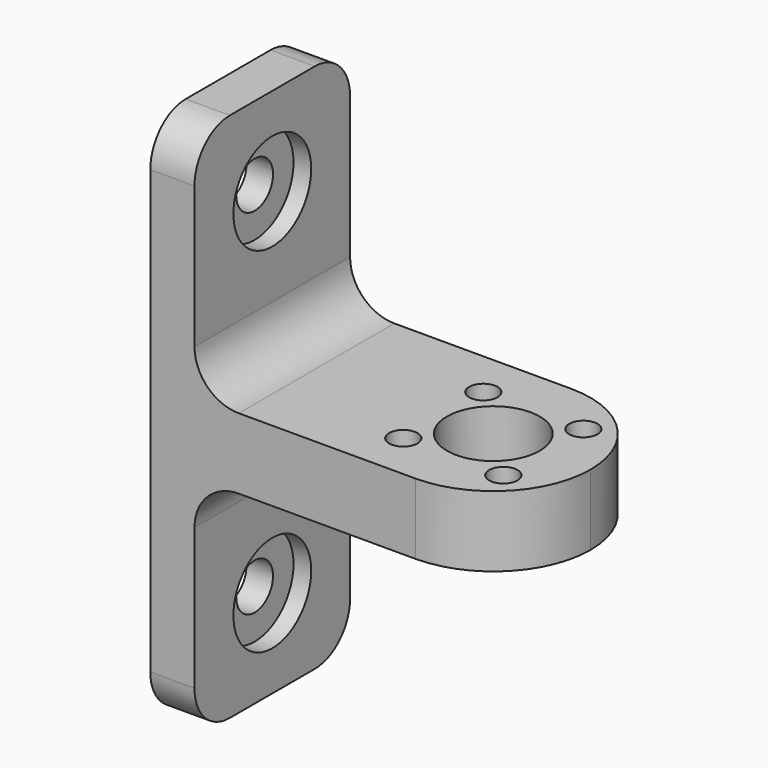
from build123d import *

# Parameters (mm, degrees)
F1_W            = 22
F1_H            = 26
F1_H_2          = 8
F2_DEPTH        = 5
F3_DEPTH        = 41
F5_D            = 10.5
F6_D            = 3.2
F7_R            = 10.99999
F8_R            = 5
F10_D           = 5.2
F10_CBORE_D     = 11
F10_CBORE_DEPTH = 2
F11_R           = 5


# Not quite as in the source:
# - a fillet or chamfer is up to 0.001 mm smaller than in the source, because OpenCascade refuses the exact size


with BuildPart() as f2:
    # F1 (on Right) → F2 (new body)
    with BuildSketch(Plane.YZ):
        with Locations((0, 17)):
            Rectangle(F1_W, F1_H)
        Rectangle(F1_W, F1_H_2)
        with Locations((0, -17)):
            Rectangle(F1_W, F1_H)
    extrude(amount=F2_DEPTH)

    # F1 (on Right) → F3 (join)
    with BuildSketch(Plane.YZ):
        Rectangle(F1_W, F1_H_2)
    extrude(amount=F3_DEPTH)

    # F5 (through all)
    with Locations(Plane.XY.offset(4)):
        with Locations((30, 0)):
            Hole(F5_D / 2)

    # F6 (through all)
    with Locations(Plane.XY.offset(4)):
        with Locations((24.3431457505, -5.6568542495), (24.3431457505, 5.6568542495), (35.6568542495, 5.6568542495), (35.6568542495, -5.6568542495)):
            Hole(F6_D / 2)

    # F7 (radius 11 in the source; OpenCascade refuses exactly that, so slightly less here)
    f7_edges = [f2.edges().sort_by_distance(p)[0] for p in [
        (41, 11, 0),
        (41, -11, 0),
    ]]
    fillet(f7_edges, radius=F7_R)

    # F8
    f8_edges = [f2.edges().sort_by_distance(p)[0] for p in [
        (5, 0, 4),
        (5, 0, -4),
    ]]
    fillet(f8_edges, radius=F8_R)

    # F10 (through all)
    with Locations(Plane.YZ.offset(5)):
        with Locations((0, 20), (0, -20)):
            CounterBoreHole(F10_D / 2, F10_CBORE_D / 2, F10_CBORE_DEPTH)

    # F11
    f11_edges = [f2.edges().sort_by_distance(p)[0] for p in [
        (2.5, -11, 30),
        (2.5, 11, 30),
        (2.5, -11, -30),
        (2.5, 11, -30),
    ]]
    fillet(f11_edges, radius=F11_R)


solid = f2.part
